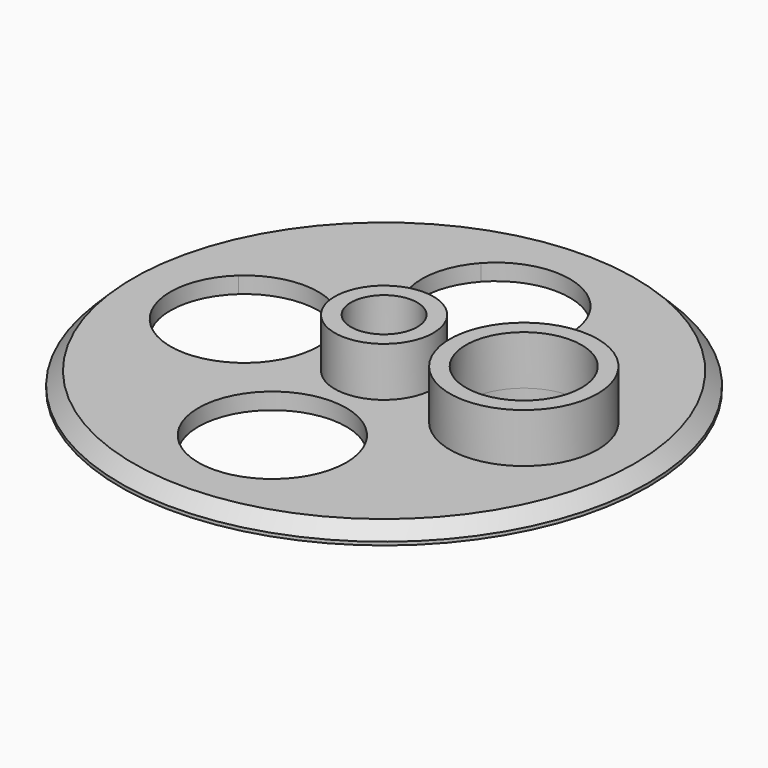
from build123d import *

# Parameters (mm, degrees)
F0_R     = 50.9905
F0_R_2   = 6.4135
F1_DEPTH = 3.175
F2_R     = 9.525
F2_R_2   = 6.4135
F2_R_3   = 14.2875
F2_R_4   = 11.176
F3_DEPTH = 9.525
F4_SIZE  = 2.54


# Not quite as in the source:
# - a feature names something its author has since deleted; it is built from what else it names


with BuildPart() as f1:
    # F0 (on Top) → F1 (new body)
    with BuildSketch(Plane.XY):
        Circle(F0_R)
        with BuildLine():
            ThreePointArc((10.565007, 36.605882), (30.017701, 23.463752), (38.073778, 1.413298))
            ThreePointArc((38.073778, 1.413298), (38.141047, 0.708071), (38.1635, 0))
            ThreePointArc((38.1635, 0), (38.141047, -0.708071), (38.073778, -1.413298))
            ThreePointArc((38.073778, -1.413298), (30.017701, -23.463752), (10.565007, -36.605882))
            ThreePointArc((10.565007, -36.605882), (0, -41.275), (-10.565007, -36.605882))
            ThreePointArc((-10.565007, -36.605882), (-26.940768, -26.940768), (-36.605882, -10.565007))
            ThreePointArc((-36.605882, -10.565007), (-41.275, 0), (-36.605882, 10.565007))
            ThreePointArc((-36.605882, 10.565007), (-26.940768, 26.940768), (-10.565007, 36.605882))
            ThreePointArc((-10.565007, 36.605882), (0, 41.275), (10.565007, 36.605882))
        make_face(mode=Mode.SUBTRACT)
        with BuildLine():
            ThreePointArc((38.073778, -1.413298), (15.8115, 0), (38.073778, 1.413298))
            ThreePointArc((38.073778, 1.413298), (30.017701, 23.463752), (10.565007, 36.605882))
            ThreePointArc((10.565007, 36.605882), (13.324417, 32.144297), (14.2875, 26.9875))
            ThreePointArc((14.2875, 26.9875), (-5.156797, 13.663083), (-10.565007, 36.605882))
            ThreePointArc((-10.565007, 36.605882), (-26.940768, 26.940768), (-36.605882, 10.565007))
            ThreePointArc((-36.605882, 10.565007), (-21.21212, 13.068192), (-12.7, 0))
            ThreePointArc((-12.7, 0), (-21.21212, -13.068192), (-36.605882, -10.565007))
            ThreePointArc((-36.605882, -10.565007), (-26.940768, -26.940768), (-10.565007, -36.605882))
            ThreePointArc((-10.565007, -36.605882), (-5.156797, -13.663083), (14.2875, -26.9875))
            ThreePointArc((14.2875, -26.9875), (13.324417, -32.144297), (10.565007, -36.605882))
            ThreePointArc((10.565007, -36.605882), (30.017701, -23.463752), (38.073778, -1.413298))
        make_face()
        Circle(F0_R_2, mode=Mode.SUBTRACT)
    extrude(amount=F1_DEPTH)

    # F2 (on face) → F3 (join)
    with BuildSketch(Plane.XY.offset(3.175)):
        Circle(F2_R)
        Circle(F2_R_2, mode=Mode.SUBTRACT)
        with Locations((26.9875, 0)):
            Circle(F2_R_3)
        with Locations((26.9875, 0)):
            Circle(F2_R_4, mode=Mode.SUBTRACT)
    extrude(amount=F3_DEPTH)

    # F4
    f4_edges = [f1.edges().sort_by_distance(p)[0] for p in [
        (-50.9905, 0, 3.175),
    ]]
    chamfer(f4_edges, length=F4_SIZE)


solid = f1.part
